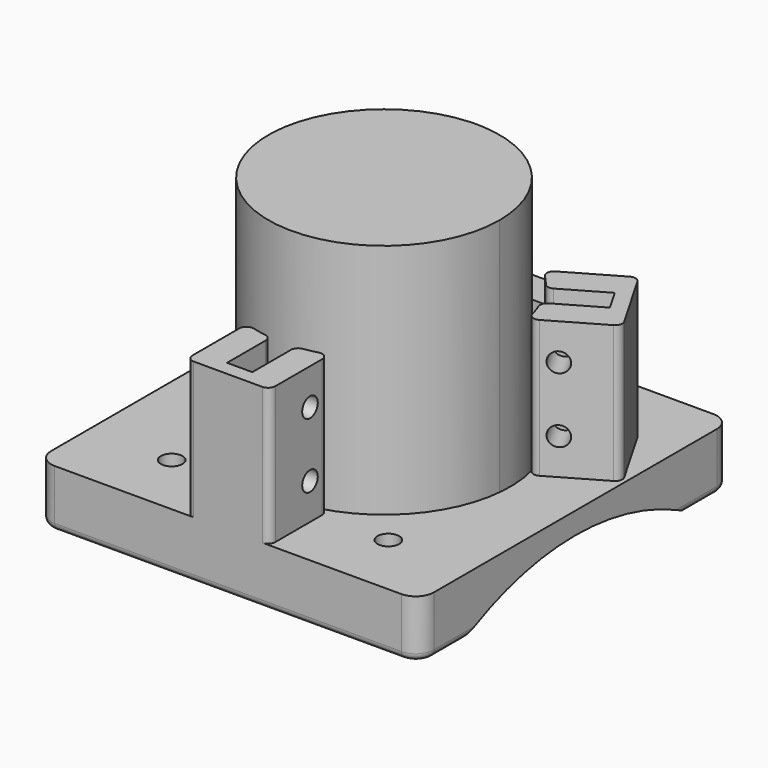
from build123d import *

# Parameters (mm, degrees)
F0_R           = 3
F1_DEPTH       = 16
F3_R           = 80
F4_DEPTH       = 500
F5_T1_DEPTH    = 15.2701665379
F5_T3_DEPTH    = 96
F5_T5_DEPTH    = 24.3208111869
F5_T7_DEPTH    = 26.3208111869
F5_T9_DEPTH    = 9.2701665379
F5_T11_DEPTH   = 10
F5_T13_DEPTH   = 26.3208111869
F5_T15_DEPTH   = 24.3208111869
F5_T17_DEPTH   = 15.2701665379
F5_T19_DEPTH   = 60.0766209806
F5_T22_ANGLE   = 90
F5_T24_ANGLE   = 90
F5_T26_ANGLE   = 240.0133105781
F5_T28_ANGLE   = 240.0133105781
F5_T30_ANGLE   = 90
F5_T32_ANGLE   = 240.0133105781
F5_T34_ANGLE   = 240.0133105781
F5_T36_ANGLE   = 90
F5_T41_DEPTH   = 15
F5_T45_DEPTH   = 14.2701665379
F5_T52_DEPTH   = 14.2701665379
F5_T56_DEPTH   = 15
F7_DEPTH       = 80
F14_COUNT      = 3
F16_DEPTH      = 38
F17_COUNT      = 3
F18_R          = 2
F18_2_R        = 2
F18_3_R        = 2
F19_R          = 2
F19_2_R        = 2
F19_3_R        = 2
F22_DEPTH      = 60
F24_DEPTH      = 18.5
F24_DEPTH_BACK = 18.5
F25_W          = 21
F25_H          = 18
F25_R          = 1.125
F26_DEPTH      = 18.926
F28_DEPTH      = 40.2010001


# Not quite as in the source:
# - a fillet or chamfer that OpenCascade refuses, or shapes differently, is made with other operations: its cross-section is extruded or revolved along the edge and cut away or added


with BuildPart() as f1:
    # F0 (on Top) → F1 (new body)
    with BuildSketch(Plane.XY):
        with BuildLine():
            Line((-48, -54), (48, -54))
            ThreePointArc((48, -54), (51.5355339059, -52.5355339059), (53, -49))
            Line((53, -49), (53, 49))
            ThreePointArc((53, 49), (51.5355339059, 52.5355339059), (48, 54))
            Line((48, 54), (-48, 54))
            ThreePointArc((-48, 54), (-51.5355339059, 52.5355339059), (-53, 49))
            Line((-53, 49), (-53, -49))
            ThreePointArc((-53, -49), (-51.5355339059, -52.5355339059), (-48, -54))
        make_face()
        with Locations((-30, -36)):
            Circle(F0_R, mode=Mode.SUBTRACT)
        with Locations((30, -36)):
            Circle(F0_R, mode=Mode.SUBTRACT)
        with Locations((-30, 36)):
            Circle(F0_R, mode=Mode.SUBTRACT)
        with BuildLine():
            ThreePointArc((5, 34.6410161514), (0, -35), (-5, 34.6410161514))
            Line((-5, 34.6410161514), (-5, 43))
            Line((-5, 43), (5, 43))
            Line((5, 43), (5, 34.6410161514))
        make_face(mode=Mode.SUBTRACT)
        with Locations((30, 36)):
            Circle(F0_R, mode=Mode.SUBTRACT)
    extrude(amount=F1_DEPTH)

    # F3 (on offset) → F4 (cut)
    with BuildSketch(Plane.YZ.offset(150)):
        with Locations((0, -70)):
            Circle(F3_R)
    extrude(amount=-F4_DEPTH, mode=Mode.SUBTRACT)

    # F5: fillet of radius 2 on 24 edges, made by hand

    # F5_s2 → F5_t1 (cut)
    with BuildSketch(Plane.XZ.offset(-49)):
        with BuildLine():
            ThreePointArc((-53, 2), (-52.4142135624, 0.5857864376), (-51, 0))
            Line((-51, 0), (-53, 0))
            Line((-53, 0), (-53, 2))
        make_face()
        with BuildLine():
            ThreePointArc((53, 2), (52.4142135624, 0.5857864376), (51, 0))
            Line((51, 0), (53, 0))
            Line((53, 0), (53, 2))
        make_face()
    extrude(amount=F5_T1_DEPTH, mode=Mode.SUBTRACT)

    # F5_s4 → F5_t3 (cut)
    with BuildSketch(Plane.YZ.offset(-48)):
        with BuildLine():
            ThreePointArc((54, 2), (53.4142135624, 0.5857864376), (52, 0))
            Line((52, 0), (54, 0))
            Line((54, 0), (54, 2))
        make_face()
        with BuildLine():
            ThreePointArc((-54, 2), (-53.4142135624, 0.5857864376), (-52, 0))
            Line((-52, 0), (-54, 0))
            Line((-54, 0), (-54, 2))
        make_face()
    extrude(amount=F5_T3_DEPTH, mode=Mode.SUBTRACT)

    # F5_s6 → F5_t5 (cut)
    with BuildSketch(Plane.YZ.offset(29.9616895097)):
        with BuildLine():
            ThreePointArc((38.2856914543, 0.243902439), (38.7489689424, 0.0619345829), (39.2428337407, 0))
            Line((39.2428337407, 0), (38.7298334621, 0))
            ThreePointArc((38.7298334621, 0), (38.5079555629, 0.1223028598), (38.2856914543, 0.243902439))
        make_face()
        with BuildLine():
            ThreePointArc((-39.2428337407, 0), (-38.7489689424, 0.0619345829), (-38.2856914543, 0.243902439))
            ThreePointArc((-38.2856914543, 0.243902439), (-38.5079555629, 0.1223028598), (-38.7298334621, 0))
            Line((-38.7298334621, 0), (-39.2428337407, 0))
        make_face()
    extrude(amount=F5_T5_DEPTH, mode=Mode.SUBTRACT)

    # F5_s8 → F5_t7 (cut)
    with BuildSketch(Plane.YZ.offset(3.7174993034)):
        with BuildLine():
            ThreePointArc((38.2856914543, 0.243902439), (38.7489689424, 0.0619345829), (39.2428337407, 0))
            Line((39.2428337407, 0), (38.7298334621, 0))
            ThreePointArc((38.7298334621, 0), (38.5079555629, 0.1223028598), (38.2856914543, 0.243902439))
        make_face()
    extrude(amount=F5_T7_DEPTH, mode=Mode.SUBTRACT)

    # F5_s10 → F5_t9 (cut)
    with BuildSketch(Plane.XZ.offset(-43)):
        with BuildLine():
            ThreePointArc((5, 2), (5.5857864376, 0.5857864376), (7, 0))
            Line((7, 0), (5, 0))
            Line((5, 0), (5, 2))
        make_face()
        with BuildLine():
            ThreePointArc((-5, 2), (-5.5857864376, 0.5857864376), (-7, 0))
            Line((-7, 0), (-5, 0))
            Line((-5, 0), (-5, 2))
        make_face()
    extrude(amount=F5_T9_DEPTH, mode=Mode.SUBTRACT)

    # F5_s12 → F5_t11 (cut)
    with BuildSketch(Plane.YZ.offset(-5)):
        with BuildLine():
            ThreePointArc((43, 2), (43.5857864376, 0.5857864376), (45, 0))
            Line((45, 0), (43, 0))
            Line((43, 0), (43, 2))
        make_face()
    extrude(amount=F5_T11_DEPTH, mode=Mode.SUBTRACT)

    # F5_s14 → F5_t13 (cut)
    with BuildSketch(Plane.YZ.offset(-30.0383104903)):
        with BuildLine():
            ThreePointArc((38.2856914543, 0.243902439), (38.7489689424, 0.0619345829), (39.2428337407, 0))
            Line((39.2428337407, 0), (38.7298334621, 0))
            ThreePointArc((38.7298334621, 0), (38.5079555629, 0.1223028598), (38.2856914543, 0.243902439))
        make_face()
    extrude(amount=F5_T13_DEPTH, mode=Mode.SUBTRACT)

    # F5_s16 → F5_t15 (cut)
    with BuildSketch(Plane.YZ.offset(-54.2825006966)):
        with BuildLine():
            ThreePointArc((38.2856914543, 0.243902439), (38.7489689424, 0.0619345829), (39.2428337407, 0))
            Line((39.2428337407, 0), (38.7298334621, 0))
            ThreePointArc((38.7298334621, 0), (38.5079555629, 0.1223028598), (38.2856914543, 0.243902439))
        make_face()
        with BuildLine():
            ThreePointArc((-39.2428337407, 0), (-38.7489689424, 0.0619345829), (-38.2856914543, 0.243902439))
            ThreePointArc((-38.2856914543, 0.243902439), (-38.5079555629, 0.1223028598), (-38.7298334621, 0))
            Line((-38.7298334621, 0), (-39.2428337407, 0))
        make_face()
    extrude(amount=F5_T15_DEPTH, mode=Mode.SUBTRACT)

    # F5_s18 → F5_t17 (cut)
    with BuildSketch(Plane.XZ.offset(33.7298334621)):
        with BuildLine():
            ThreePointArc((-51, 0), (-52.4142135624, 0.5857864376), (-53, 2))
            Line((-53, 2), (-53, 0))
            Line((-53, 0), (-51, 0))
        make_face()
        with BuildLine():
            ThreePointArc((51, 0), (52.4142135624, 0.5857864376), (53, 2))
            Line((53, 2), (53, 0))
            Line((53, 0), (51, 0))
        make_face()
    extrude(amount=F5_T17_DEPTH, mode=Mode.SUBTRACT)

    # F5_s20 → F5_t19 (cut)
    with BuildSketch(Plane.YZ.offset(-30.0383104903)):
        with BuildLine():
            ThreePointArc((-39.2428337407, 0), (-38.7489689424, 0.0619345829), (-38.2856914543, 0.243902439))
            ThreePointArc((-38.2856914543, 0.243902439), (-38.5079555629, 0.1223028598), (-38.7298334621, 0))
            Line((-38.7298334621, 0), (-39.2428337407, 0))
        make_face()
    extrude(amount=F5_T19_DEPTH, mode=Mode.SUBTRACT)

    # F5_s21 → F5_t22 (revolve, cut)
    with BuildSketch(Plane.YZ.offset(-48)):
        with BuildLine():
            ThreePointArc((54, 2), (53.4142135624, 0.5857864376), (52, 0))
            Line((52, 0), (54, 0))
            Line((54, 0), (54, 2))
        make_face()
    revolve(axis=Axis((-48, 49, 0), (0, 0, 1)), revolution_arc=F5_T22_ANGLE, mode=Mode.SUBTRACT)

    # F5_s23 → F5_t24 (revolve, cut)
    with BuildSketch(Plane.XZ.offset(-49)):
        with BuildLine():
            ThreePointArc((53, 2), (52.4142135624, 0.5857864376), (51, 0))
            Line((51, 0), (53, 0))
            Line((53, 0), (53, 2))
        make_face()
    revolve(axis=Axis((48, 49, 0), (0, 0, 1)), revolution_arc=F5_T24_ANGLE, mode=Mode.SUBTRACT)

    # F5_s25 → F5_t26 (revolve, cut)
    with BuildSketch(Plane(origin=(23.0935657103, 39.9885014063, 0), x_dir=(0, 0, 1), z_dir=(-0.5001005913, -0.8659673196, 0))):
        with BuildLine():
            ThreePointArc((2, -10.9753983014), (0.5857864376, -11.561184739), (0, -12.9753983014))
            Line((0, -12.9753983014), (0, -10.9753983014))
            Line((0, -10.9753983014), (2, -10.9753983014))
        make_face()
    revolve(axis=Axis((30, 36, 0), (0, 0, 1)), revolution_arc=F5_T26_ANGLE, mode=Mode.SUBTRACT)

    # F5_s27 → F5_t28 (revolve, cut)
    with BuildSketch(Plane(origin=(8.087529626, 14.0042552927, 0), x_dir=(0, 0, 1), z_dir=(-0.5001005913, -0.8659673196, 0))):
        with BuildLine():
            ThreePointArc((2, 40.9826408739), (0.5857864376, 40.3968544363), (0, 38.9826408739))
            Line((0, 38.9826408739), (0, 40.9826408739))
            Line((0, 40.9826408739), (2, 40.9826408739))
        make_face()
    revolve(axis=Axis((-30, 36, 0), (0, 0, 1)), revolution_arc=F5_T28_ANGLE, mode=Mode.SUBTRACT)

    # F5_s29 → F5_t30 (revolve, cut)
    with BuildSketch(Plane.XZ.offset(49)):
        with BuildLine():
            ThreePointArc((-53, 2), (-52.4142135624, 0.5857864376), (-51, 0))
            Line((-51, 0), (-53, 0))
            Line((-53, 0), (-53, 2))
        make_face()
    revolve(axis=Axis((-48, -49, 0), (0, 0, 1)), revolution_arc=F5_T30_ANGLE, mode=Mode.SUBTRACT)

    # F5_s31 → F5_t32 (revolve, cut)
    with BuildSketch(Plane(origin=(-23.0935657103, -39.9885014063, 0), x_dir=(0, 0, 1), z_dir=(0.5001005913, 0.8659673196, 0))):
        with BuildLine():
            ThreePointArc((0, -12.9753983014), (0.5857864376, -11.561184739), (2, -10.9753983014))
            Line((2, -10.9753983014), (0, -10.9753983014))
            Line((0, -10.9753983014), (0, -12.9753983014))
        make_face()
    revolve(axis=Axis((-30, -36, 0), (0, 0, 1)), revolution_arc=F5_T32_ANGLE, mode=Mode.SUBTRACT)

    # F5_s33 → F5_t34 (revolve, cut)
    with BuildSketch(Plane(origin=(-8.087529626, -14.0042552927, 0), x_dir=(0, 0, 1), z_dir=(0.5001005913, 0.8659673196, 0))):
        with BuildLine():
            ThreePointArc((0, 38.9826408739), (0.5857864376, 40.3968544363), (2, 40.9826408739))
            Line((2, 40.9826408739), (0, 40.9826408739))
            Line((0, 40.9826408739), (0, 38.9826408739))
        make_face()
    revolve(axis=Axis((30, -36, 0), (0, 0, 1)), revolution_arc=F5_T34_ANGLE, mode=Mode.SUBTRACT)

    # F5_s35 → F5_t36 (revolve, cut)
    with BuildSketch(Plane.YZ.offset(48)):
        with BuildLine():
            ThreePointArc((-54, 2), (-53.4142135624, 0.5857864376), (-52, 0))
            Line((-52, 0), (-54, 0))
            Line((-54, 0), (-54, 2))
        make_face()
    revolve(axis=Axis((48, -49, 0), (0, 0, 1)), revolution_arc=F5_T36_ANGLE, mode=Mode.SUBTRACT)


with BuildPart() as f5_tool39:
    # F5_s40 → F5_t41 (new body)
    with BuildSketch(Plane.YZ.offset(-5)):
        with BuildLine():
            ThreePointArc((43, 2), (43.5857864376, 0.5857864376), (45, 0))
            Line((45, 0), (43, 0))
            Line((43, 0), (43, 2))
        make_face()
    extrude(amount=F5_T41_DEPTH)

    split(bisect_by=Plane.YZ.offset(5), keep=Keep.TOP)


with BuildPart() as f5_tool43:
    # F5_s44 → F5_t45 (new body)
    with BuildSketch(Plane.XZ.offset(-48)):
        with BuildLine():
            ThreePointArc((5, 2), (5.5857864376, 0.5857864376), (7, 0))
            Line((7, 0), (5, 0))
            Line((5, 0), (5, 2))
        make_face()
    extrude(amount=F5_T45_DEPTH)

    split(bisect_by=Plane.XZ.offset(-43), keep=Keep.BOTTOM)


with BuildPart() as f5_tool39_1:
    add(f5_tool39.part)

    # F5_t47: intersect F5_tool43
    add(f5_tool43.part, mode=Mode.INTERSECT)


with BuildPart() as f1_1:
    add(f1.part)

    # F5_t37: cut F5_tool39
    add(f5_tool39_1.part, mode=Mode.SUBTRACT)


with BuildPart() as f5_tool50:
    # F5_s51 → F5_t52 (new body)
    with BuildSketch(Plane.XZ.offset(-33.7298334621)):
        with BuildLine():
            ThreePointArc((-5, 2), (-5.5857864376, 0.5857864376), (-7, 0))
            Line((-7, 0), (-5, 0))
            Line((-5, 0), (-5, 2))
        make_face()
    extrude(amount=-F5_T52_DEPTH)

    split(bisect_by=Plane.XZ.offset(-43), keep=Keep.BOTTOM)


with BuildPart() as f5_tool54:
    # F5_s55 → F5_t56 (new body)
    with BuildSketch(Plane.YZ.offset(-10)):
        with BuildLine():
            ThreePointArc((43, 2), (43.5857864376, 0.5857864376), (45, 0))
            Line((45, 0), (43, 0))
            Line((43, 0), (43, 2))
        make_face()
    extrude(amount=F5_T56_DEPTH)

    split(bisect_by=Plane.YZ.offset(-5), keep=Keep.BOTTOM)


with BuildPart() as f5_tool50_1:
    add(f5_tool50.part)

    # F5_t58: intersect F5_tool54
    add(f5_tool54.part, mode=Mode.INTERSECT)


with BuildPart() as f1_2:
    add(f1_1.part)

    # F5_t48: cut F5_tool50
    add(f5_tool50_1.part, mode=Mode.SUBTRACT)


with BuildPart() as f7:
    # F6 (on Top) → F7 (new body)
    with BuildSketch(Plane.XY):
        with BuildLine():
            ThreePointArc((-2, 31.9374388453), (-21.9089023002, -23.3238075794), (32, 0))
            ThreePointArc((32, 0), (23.3238075794, 21.9089023002), (2, 31.9374388453))
            ThreePointArc((2, 31.9374388453), (0, 32), (-2, 31.9374388453))
        make_face()
    extrude(amount=F7_DEPTH)

    # F6 (on Top) → F22 (join)
    with BuildSketch(Plane.XY):
        with BuildLine():
            ThreePointArc((-2, 31.9374388453), (-21.9089023002, -23.3238075794), (32, 0))
            ThreePointArc((32, 0), (23.3238075794, 21.9089023002), (2, 31.9374388453))
            ThreePointArc((2, 31.9374388453), (0, 32), (-2, 31.9374388453))
        make_face()
        with BuildLine():
            ThreePointArc((-2, 31.9374388453), (0, 32), (2, 31.9374388453))
            Line((2, 31.9374388453), (2, 34.7))
            Line((2, 34.7), (0, 34.7))
            Line((0, 34.7), (-2, 34.7))
            Line((-2, 34.7), (-2, 31.9374388453))
        make_face()
    extrude(amount=F22_DEPTH)


with BuildPart() as f12:
    # F11 (on offset) → F12 (revolve)
    with BuildSketch(Plane.XY.offset(44)):
        Polygon((2.5, -32), (0, -32), (-2.5, -32), (-2.5, -37.3), (-12.4999610707, -37.3), (-12.4999610707, -40), (12.5000389293, -40), (12.5000389293, -37.3), (2.5, -37.3), align=None)
    revolve(axis=Axis((3.89293e-05, -40, 44), (-1, 0, 0)))


with BuildPart() as f13:
    # F9 (on offset) → F13 (revolve)
    with BuildSketch(Plane.XY.offset(26)):
        Polygon((2.5, -32), (0, -32), (-2.5, -32), (-2.5, -37.3), (-12.5, -37.3), (-12.5, -40), (12.5, -40), (12.5, -37.3), (2.5, -37.3), align=None)
    revolve(axis=Axis((0, -40, 26), (1, 0, 0)))


with BuildPart() as f14_1:
    # F14: instance of F13
    add(f13.part.rotate(Axis((0, 0, 0), (0, 0, -1)), 1 * 360 / F14_COUNT))


with BuildPart() as f14_2:
    # F14: instance of F13
    add(f13.part.rotate(Axis((0, 0, 0), (0, 0, -1)), 2 * 360 / F14_COUNT))


with BuildPart() as f14_3:
    # F14: instance of F12
    add(f12.part.rotate(Axis((0, 0, 0), (0, 0, -1)), 1 * 360 / F14_COUNT))


with BuildPart() as f14_4:
    # F14: instance of F12
    add(f12.part.rotate(Axis((0, 0, 0), (0, 0, -1)), 2 * 360 / F14_COUNT))


with BuildPart() as f16:
    # F15 (on face) → F16 (new body)
    with BuildSketch(Plane.XY.offset(16)):
        with BuildLine():
            Line((-11.5, -54), (0, -54))
            Line((0, -54), (0, -49.9654337764))
            Line((0, -49.9654337764), (-3.5, -49.9654337764))
            Line((-3.5, -49.9654337764), (-3.5, -34.8245602987))
            ThreePointArc((-3.5, -34.8245602987), (-7.5519051376, -34.175557476), (-11.5, -33.0567693521))
            Line((-11.5, -33.0567693521), (-11.5, -54))
        make_face()
        with BuildLine():
            Line((0, -49.9654337764), (0, -54))
            Line((0, -54), (11.5, -54))
            Line((11.5, -54), (11.5, -33.0567693521))
            ThreePointArc((11.5, -33.0567693521), (7.5519051376, -34.175557476), (3.5, -34.8245602987))
            Line((3.5, -34.8245602987), (3.5, -49.9654337764))
            Line((3.5, -49.9654337764), (0, -49.9654337764))
        make_face()
    extrude(amount=F16_DEPTH)


with BuildPart() as f17_1:
    # F17: instance of F16
    add(f16.part.rotate(Axis((0, 0, 0), (0, 0, -1)), 1 * 360 / F17_COUNT))

    # F18#2
    f18_2_edges = [f17_1.edges().sort_by_distance(p)[0] for p in [
        (-22.878002, 26.487677, 35),
        (-41.015372, 36.959292, 35),
        (-52.515372, 17.040708, 35),
        (-34.378002, 6.569093, 35),
    ]]
    fillet(f18_2_edges, radius=F18_2_R)

    # F19
    f19_edges = [f17_1.edges().sort_by_distance(p)[0] for p in [
        (-28.408954, 20.443369, 35),
        (-31.908954, 14.381191, 35),
    ]]
    fillet(f19_edges, radius=F19_R)


with BuildPart() as f17_2:
    # F17: instance of F16
    add(f16.part.rotate(Axis((0, 0, 0), (0, 0, -1)), 2 * 360 / F17_COUNT))

    # F18
    f18_edges = [f17_2.edges().sort_by_distance(p)[0] for p in [
        (52.515372, 17.040708, 35),
        (41.015372, 36.959292, 35),
        (22.878002, 26.487677, 35),
        (34.378002, 6.569093, 35),
    ]]
    fillet(f18_edges, radius=F18_R)

    # F19#2
    f19_2_edges = [f17_2.edges().sort_by_distance(p)[0] for p in [
        (31.908954, 14.381191, 35),
        (28.408954, 20.443369, 35),
    ]]
    fillet(f19_2_edges, radius=F19_2_R)


with BuildPart() as f16_1:
    add(f16.part)

    # F18#3
    f18_3_edges = [f16_1.edges().sort_by_distance(p)[0] for p in [
        (11.5, -33.056769, 35),
        (11.5, -54, 35),
        (-11.5, -54, 35),
        (-11.5, -33.056769, 35),
    ]]
    fillet(f18_3_edges, radius=F18_3_R)

    # F19#3
    f19_3_edges = [f16_1.edges().sort_by_distance(p)[0] for p in [
        (3.5, -34.82456, 35),
        (-3.5, -34.82456, 35),
    ]]
    fillet(f19_3_edges, radius=F19_3_R)


with BuildPart() as f17_2_1:
    add(f17_2.part)

    # F20: union F17_1, F16, F1
    add(f17_1.part)
    add(f16_1.part)
    add(f1_2.part)

    # F21: cut F14_2, F14_1, F13, F12, F14_3, F14_4
    add(f14_2.part, mode=Mode.SUBTRACT)
    add(f14_1.part, mode=Mode.SUBTRACT)
    add(f13.part, mode=Mode.SUBTRACT)
    add(f12.part, mode=Mode.SUBTRACT)
    add(f14_3.part, mode=Mode.SUBTRACT)
    add(f14_4.part, mode=Mode.SUBTRACT)


with BuildPart() as f24:
    # F23 (on Right) → F24 (new body, two sides)
    with BuildSketch(Plane.YZ) as f24_sk:
        with BuildLine():
            Line((36.7, 28.6), (35.075, 28.6))
            Line((35.075, 28.6), (35.075, 17))
            Line((35.075, 17), (44.2, 17))
            Line((44.2, 17), (44.2, 26))
            Line((44.2, 26), (39.3, 26))
            ThreePointArc((39.3, 26), (37.4615223689, 26.7615223689), (36.7, 28.6))
        make_face()
        with BuildLine():
            Line((44.2, 40.2), (35.075, 40.2))
            Line((35.075, 40.2), (35.075, 28.6))
            Line((35.075, 28.6), (36.7, 28.6))
            ThreePointArc((36.7, 28.6), (37.4615223689, 30.4384776311), (39.3, 31.2))
            Line((39.3, 31.2), (44.2, 31.2))
            Line((44.2, 31.2), (44.2, 40.2))
        make_face()
    extrude(amount=F24_DEPTH)
    extrude(f24_sk.sketch, amount=-F24_DEPTH_BACK)

    # F25 (on face) → F26 (cut, through all)
    with BuildSketch(Plane.XZ.offset(-35.075)):
        with Locations((0, 28.6)):
            Rectangle(F25_W, F25_H)
        with Locations((-14, 35.35)):
            Circle(F25_R)
        with Locations((14, 35.35)):
            Circle(F25_R)
        with Locations((14, 21.85)):
            Circle(F25_R)
        with Locations((-14, 21.85)):
            Circle(F25_R)
    extrude(amount=-F26_DEPTH, mode=Mode.SUBTRACT)

    # F27 (on face) → F28 (cut, through all)
    with BuildSketch(Plane.XY.offset(40.2)):
        Polygon((-2.5, 35.075), (0, 35.075), (2.5, 35.075), (2.5, 38.075), (-2.5, 38.075), align=None)
    extrude(amount=-F28_DEPTH, mode=Mode.SUBTRACT)


solid = Compound([f7.part, f17_2_1.part, f24.part])
